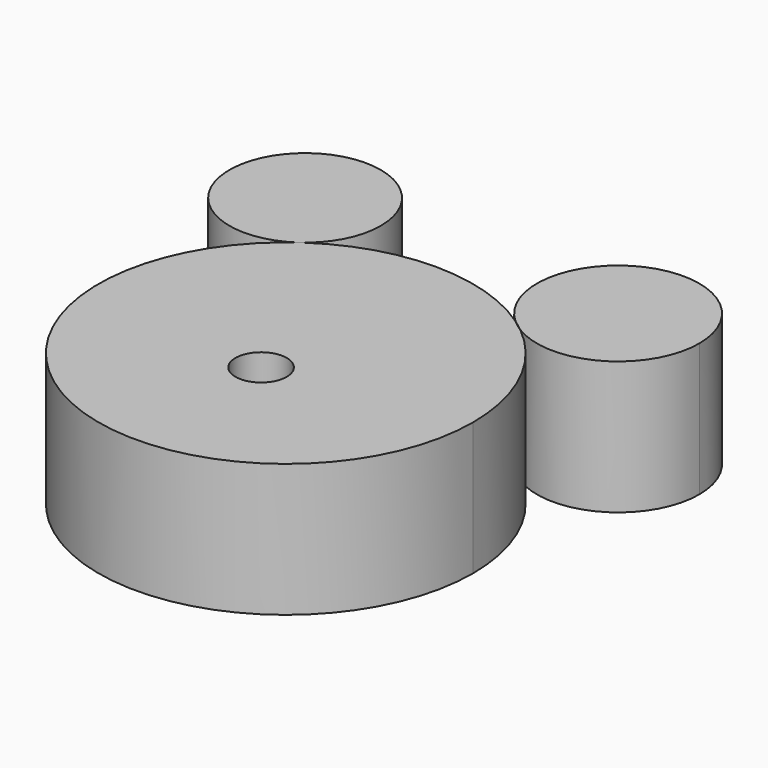
from build123d import *

# Parameters (mm, degrees)
F0_R     = 4.8983295198
F1_DEPTH = 25.4
F0_R_2   = 14.4664110347


# Not quite as in the source:
# - the program builds the solid bodies; features that only make, move or delete a surface that nothing else refers to are left out


with BuildPart() as f1:
    # F0 (on Top) → F1 (new body)
    with BuildSketch(Plane.XY):
        with BuildLine():
            ThreePointArc((20.3225355866, 29.4635993727), (-31.6899449587, -16.6390062557), (35.7925849956, 0))
            ThreePointArc((35.7925849956, 0), (32.3182399262, 15.3831241541), (22.5697060798, 27.7798039614))
            ThreePointArc((22.5697060798, 27.7798039614), (21.4079475638, 28.5707561401), (20.3225355866, 29.4635993727))
        make_face()
        with Locations((0, -5.8903987519)):
            Circle(F0_R, mode=Mode.SUBTRACT)
    extrude(amount=F1_DEPTH)


with BuildPart() as f1b:
    # F0 (on Top) → F1, piece 2 (new body)
    with BuildSketch(Plane.XY):
        with Locations((-29.0945470333, 40.9863628447)):
            Circle(F0_R_2)
    extrude(amount=F1_DEPTH)


with BuildPart() as f1c:
    # F0 (on Top) → F1, piece 3 (new body)
    with BuildSketch(Plane.XY):
        with BuildLine():
            ThreePointArc((20.3225355866, 29.4635993727), (21.4626394122, 28.6437471383), (22.5697060798, 27.7798039614))
            ThreePointArc((22.5697060798, 27.7798039614), (38.2735681299, 27.440197867), (46.2251736271, 40.9863628447))
            ThreePointArc((46.2251736271, 40.9863628447), (24.4051814016, 55.1613472846), (20.3225355866, 29.4635993727))
        make_face()
    extrude(amount=F1_DEPTH)


solid = Compound([f1.part, f1b.part, f1c.part])
